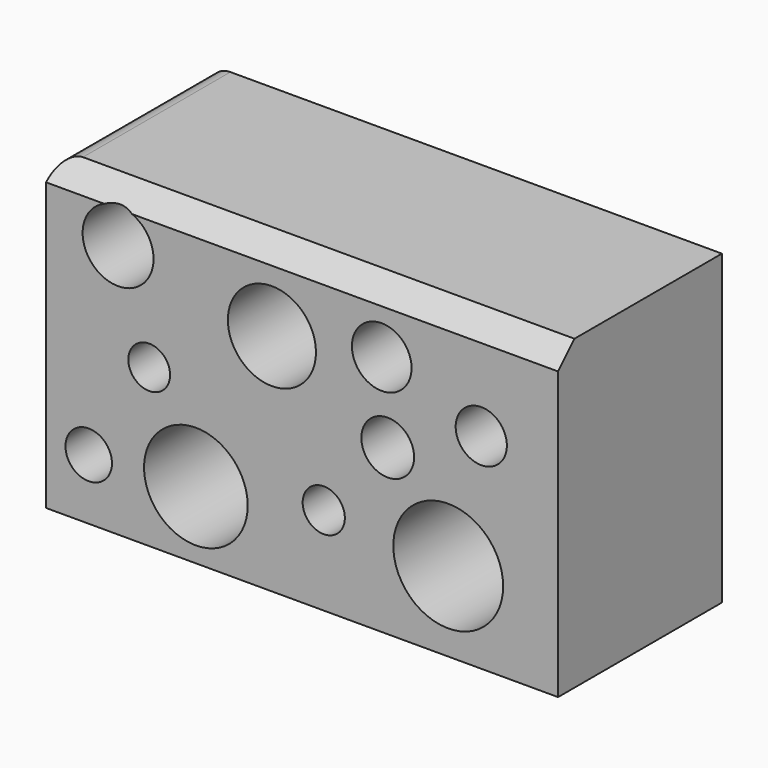
from build123d import *

# Parameters (mm, degrees)
F0_W        = 127
F0_H        = 76.2
F0_R        = 5.7659781113
F0_R_2      = 12.8582731401
F0_R_3      = 5.2319601114
F0_R_4      = 13.6233305285
F0_R_5      = 5.1796195503
F0_R_6      = 10.9267536549
F0_R_7      = 8.7936415442
F0_R_8      = 6.5428428961
F0_R_9      = 6.35
F1_DEPTH    = 50.8
F2_R        = 7.4007288491
F3_DEPTH    = 51.054
F4_T1_DEPTH = 153.1282991577
F5_R        = 5.08


# Not quite as in the source:
# - a fillet or chamfer that OpenCascade refuses, or shapes differently, is made with other operations: its cross-section is extruded or revolved along the edge and cut away or added


with BuildPart() as f1:
    # F0 (on Front) → F1 (new body)
    with BuildSketch(Plane.XZ):
        with Locations((1.9998494536, 3.723031328)):
            Rectangle(F0_W, F0_H)
        with Locations((-50.9259700775, -19.3260908127)):
            Circle(F0_R, mode=Mode.SUBTRACT)
        with Locations((-24.3451949209, -17.612459138)):
            Circle(F0_R_2, mode=Mode.SUBTRACT)
        with Locations((7.3802489787, -12.4715631828)):
            Circle(F0_R_3, mode=Mode.SUBTRACT)
        with Locations((38.248244673, -14.6136032417)):
            Circle(F0_R_4, mode=Mode.SUBTRACT)
        with Locations((-35.9206944704, 4.664753098)):
            Circle(F0_R_5, mode=Mode.SUBTRACT)
        with Locations((-5.4814172909, 21.3726628572)):
            Circle(F0_R_6, mode=Mode.SUBTRACT)
        with Locations((-43.6376929283, 28.6555960774)):
            Circle(F0_R_7, mode=Mode.SUBTRACT)
        with Locations((23.2429709285, 6.3783847727)):
            Circle(F0_R_8, mode=Mode.SUBTRACT)
        with Locations((46.4498494536, 16.423031328)):
            Circle(F0_R_9, mode=Mode.SUBTRACT)
    extrude(amount=F1_DEPTH)

    # F2 (on face) → F3 (cut)
    with BuildSketch(Plane.XZ.offset(50.8)):
        with Locations((21.7594634742, 25.6567392498)):
            Circle(F2_R)
    extrude(amount=-F3_DEPTH, mode=Mode.SUBTRACT)

    # F4: chamfer of 5.08 on 1 edges, made by hand

    # F4_s2 → F4_t1 (cut)
    with BuildSketch(Plane.YZ.offset(-74.5643001253)):
        Polygon((-45.72, 41.823031328), (-50.8, 36.743031328), (-50.8, 41.823031328), align=None)
    extrude(amount=F4_T1_DEPTH, mode=Mode.SUBTRACT)

    # F5
    f5_edges = [f1.edges().sort_by_distance(p)[0] for p in [
        (-61.500151, -22.86, 41.823031),
    ]]
    fillet(f5_edges, radius=F5_R)


solid = f1.part
